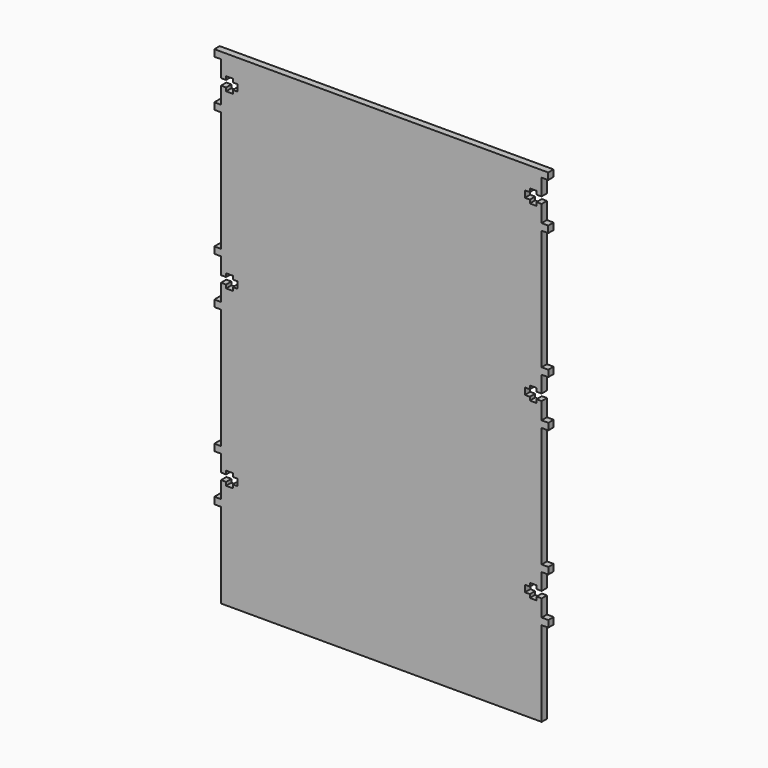
from build123d import *

# Parameters (mm, degrees)
F1_DEPTH = 3.175


# Not quite as in the source:
# - ends of sketch curves that miss each other by under 0.0002 mm in the source are joined


with BuildPart() as f1:
    # F0 (on Front) → F1 (new body)
    with BuildSketch(Plane.XZ):
        Polygon((-0.0247448797, 196.3262024198), (-79.3997448797, 196.3262024198), (-79.3997448797, 193.1512024198), (-76.2247448797, 193.1512024198), (-76.2247448797, 185.2391024198), (-73.8117448797, 185.2391024198), (-73.8117448797, 186.8520024198), (-70.6367448797, 186.8520024198), (-70.6367448797, 185.2391024198), (-68.2745449228, 185.2899024198), (-68.2745449228, 182.1149024198), (-70.6367449228, 182.1149024198), (-70.6367449228, 180.5020024198), (-73.8117449228, 180.5020024198), (-73.8117449228, 182.1149024198), (-76.2247448797, 182.1149024198), (-76.2247448797, 174.1012024198), (-79.3997448797, 174.1012024198), (-79.3997448797, 170.9262024198), (-76.2247448797, 170.9262024198), (-76.2247448797, 113.7762024198), (-79.3997448797, 113.7762024198), (-79.3997421861, 110.6520024198), (-76.2247421861, 110.6520024198), (-76.2247421861, 102.7399024198), (-73.8117421861, 102.7399024198), (-73.8117421861, 104.3528024198), (-70.6367421861, 104.3528024198), (-70.6367421861, 102.7399024198), (-68.2745421861, 102.7907024198), (-68.2745421861, 99.6157024198), (-70.6367421861, 99.6157024198), (-70.6367421861, 98.0028024198), (-73.8117421861, 98.0028024198), (-73.8117421861, 99.6157024198), (-76.2247421861, 99.6157024198), (-76.2247421861, 91.5512024198), (-79.3997421861, 91.5512024198), (-79.3997421861, 88.3762024198), (-76.2247449228, 88.3762024198), (-76.2247449228, 31.2262024198), (-79.3997448797, 31.2262024198), (-79.3997421861, 28.0512024198), (-76.2247421861, 28.0512024198), (-76.2247421861, 20.1391024198), (-73.8117421861, 20.1391024198), (-73.8117421861, 21.7520024198), (-70.6367421861, 21.7520024198), (-70.6367421861, 20.1391024198), (-68.2745421861, 20.1899024198), (-68.2745421861, 17.0149024198), (-70.6367421861, 17.0149024198), (-70.6367421861, 15.4020024198), (-73.8117421861, 15.4020024198), (-73.8117421861, 17.0149024198), (-76.2247421861, 17.0149024198), (-76.2247421861, 9.0012024198), (-79.3997421861, 9.0012024198), (-79.3997421861, 5.8262024198), (-76.2247421861, 5.8262024198), (-76.2247421861, -34.6613975802), (0, -34.6613975802), align=None)
        Polygon((79.3502532985, 196.3432087423), (-0.0247448797, 196.3262024198), (0, -34.6613975802), (76.2247404365, -34.6450662095), (76.2160658516, 5.8425328612), (79.3910657787, 5.8432131141), (79.3903855258, 9.0182130412), (76.2153855987, 9.0175327883), (76.2136686404, 17.0312326044), (73.8006686958, 17.0307156122), (73.8010142642, 15.4178156492), (70.6260143371, 15.4171353963), (70.6256687686, 17.0300353593), (68.2634688228, 17.0295292511), (68.2627885699, 20.2045291783), (70.6249993998, 20.1542352876), (70.6246538313, 21.7671352506), (73.7996537584, 21.7678155035), (73.7999993269, 20.1549155405), (76.2129992715, 20.1554325327), (76.2113040813, 28.0675323511), (79.3863040084, 28.068212604), (79.3856264492, 31.2432125317), (76.2106265651, 31.2425322788), (76.198382013, 88.3925309671), (79.3733792034, 88.3932112194), (79.3726989505, 91.5682111465), (76.1976990233, 91.5675308936), (76.195971181, 99.6320307085), (73.7829712364, 99.6315137163), (73.7833168048, 98.0186137533), (70.6083168777, 98.0179335004), (70.6079713092, 99.6308334634), (68.2457713634, 99.6303273553), (68.2450911105, 102.8053272824), (70.6073019404, 102.7550333917), (70.6069563719, 104.3679333547), (73.781956299, 104.3686136076), (73.7823018675, 102.7557136446), (76.1953018121, 102.7562306368), (76.1936066219, 110.6683304552), (79.368606549, 110.6690107081), (79.3679371802, 113.7932106364), (76.1929399467, 113.7925303841), (76.1806953945, 170.9425290724), (79.3556953216, 170.9432093253), (79.3550150687, 174.1182092524), (76.1800151416, 174.1175289995), (76.1782981833, 182.1312288156), (73.7652982818, 182.1307118234), (73.7656438503, 180.5178118604), (70.5906439231, 180.5171316075), (70.5902983547, 182.1300315705), (68.2280984089, 182.1295254623), (68.227418156, 185.3045253894), (70.5896289427, 185.2542314987), (70.5892833742, 186.8671314617), (73.7642833014, 186.8678117146), (73.7646288698, 185.2549117516), (76.1776288145, 185.2554287439), (76.1759336242, 193.1675285623), (79.3509335514, 193.1682088151), align=None)
    extrude(amount=F1_DEPTH)


solid = f1.part
